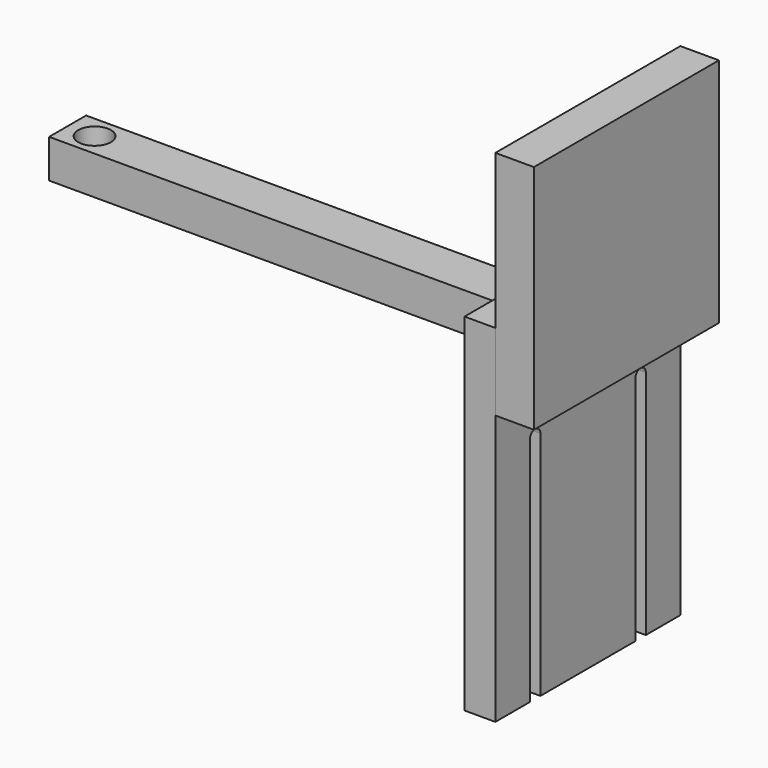
from build123d import *

# Parameters (mm, degrees)
F0_W     = 135
F0_H     = 12
F0_R     = 4.25
F1_DEPTH = 10
F0_W_2   = 5
F2_DEPTH = 60
F4_DEPTH = 5
F5_DEPTH = 3


with BuildPart() as f1:
    # F0 (on Top) → F1 (new body)
    with BuildSketch(Plane.XY):
        with Locations((-2.5, 0)):
            Rectangle(F0_W, F0_H)
        with Locations((-63, 0)):
            Circle(F0_R, mode=Mode.SUBTRACT)
    extrude(amount=F1_DEPTH)

    # F0 (on Top) → F2 (join)
    with BuildSketch(Plane.XY):
        Polygon((65, 30), (65, 6), (70, 6), (70, -6), (65, -6), (65, -30), (75, -30), (75, 30), align=None)
        with Locations((67.5, 0)):
            Rectangle(F0_W_2, F0_H)
    extrude(amount=F2_DEPTH)


with BuildPart() as f4:
    # F3 (on face) → F4 (new body)
    with BuildSketch(Plane(origin=(65, 0, 0), x_dir=(0, -1, 0), z_dir=(-1, 0, 0))):
        with BuildLine():
            Line((-6, 0), (-30, 0))
            Line((-30, 0), (-30, -70))
            Line((-30, -70), (-20, -70))
            Line((-20, -70), (-20, -10))
            ThreePointArc((-20, -10), (-17.1, -7.1), (-14.2, -10))
            Line((-14.2, -10), (-14.2, -70))
            Line((-14.2, -70), (14.2, -70))
            Line((14.2, -70), (14.2, -10))
            ThreePointArc((14.2, -10), (17.1, -7.1), (20, -10))
            Line((20, -10), (20, -70))
            Line((20, -70), (30, -70))
            Line((30, -70), (30, 0))
            Line((30, 0), (6, 0))
            Line((6, 0), (-6, 0))
        make_face()
        Polygon((-30, 20), (-30, 0), (-6, 0), (-6, 10), (-6, 20), align=None)
        Polygon((6, 10), (6, 0), (30, 0), (30, 20), (6, 20), align=None)
    extrude(amount=F4_DEPTH)

    # F3 (on face) + F4_face (on face) + F4_face1 (on face) → F5 (join)
    with BuildSketch(Plane(origin=(65, 0, 0), x_dir=(0, -1, 0), z_dir=(-1, 0, 0))):
        with BuildLine():
            Line((-20, -10), (-20, -70))
            Line((-20, -70), (-18.8, -70))
            Line((-18.8, -70), (-18.8, -10))
            ThreePointArc((-18.8, -10), (-17.1, -8.3), (-15.4, -10))
            Line((-15.4, -10), (-15.4, -70))
            Line((-15.4, -70), (-14.2, -70))
            Line((-14.2, -70), (-14.2, -10))
            ThreePointArc((-14.2, -10), (-17.1, -7.1), (-20, -10))
        make_face()
        with BuildLine():
            Line((18.8, -70), (20, -70))
            Line((20, -70), (20, -10))
            ThreePointArc((20, -10), (17.1, -7.1), (14.2, -10))
            Line((14.2, -10), (14.2, -70))
            Line((14.2, -70), (15.4, -70))
            Line((15.4, -70), (15.4, -10))
            ThreePointArc((15.4, -10), (17.1, -8.3), (18.8, -10))
            Line((18.8, -10), (18.8, -70))
        make_face()
        with BuildLine():
            Line((-6, 0), (-30, 0))
            Line((-30, 0), (-30, -70))
            Line((-30, -70), (-20, -70))
            Line((-20, -70), (-20, -10))
            ThreePointArc((-20, -10), (-17.1, -7.1), (-14.2, -10))
            Line((-14.2, -10), (-14.2, -70))
            Line((-14.2, -70), (14.2, -70))
            Line((14.2, -70), (14.2, -10))
            ThreePointArc((14.2, -10), (17.1, -7.1), (20, -10))
            Line((20, -10), (20, -70))
            Line((20, -70), (30, -70))
            Line((30, -70), (30, 0))
            Line((30, 0), (6, 0))
            Line((6, 0), (-6, 0))
        make_face()
    with BuildSketch(Plane(origin=(60, 0, -24.6369260479), x_dir=(0, -1, 0), z_dir=(-1, 0, 0))):
        with BuildLine():
            Line((20, 14.6369260479), (20, -45.3630739521))
            Line((20, -45.3630739521), (30, -45.3630739521))
            Line((30, -45.3630739521), (30, 44.6369260479))
            Line((30, 44.6369260479), (6, 44.6369260479))
            Line((6, 44.6369260479), (6, 24.6369260479))
            Line((6, 24.6369260479), (-6, 24.6369260479))
            Line((-6, 24.6369260479), (-6, 44.6369260479))
            Line((-6, 44.6369260479), (-30, 44.6369260479))
            Line((-30, 44.6369260479), (-30, -45.3630739521))
            Line((-30, -45.3630739521), (-20, -45.3630739521))
            Line((-20, -45.3630739521), (-20, 14.6369260479))
            ThreePointArc((-20, 14.6369260479), (-17.1, 17.5369260479), (-14.2, 14.6369260479))
            Line((-14.2, 14.6369260479), (-14.2, -45.3630739521))
            Line((-14.2, -45.3630739521), (14.2, -45.3630739521))
            Line((14.2, -45.3630739521), (14.2, 14.6369260479))
            ThreePointArc((14.2, 14.6369260479), (17.1, 17.5369260479), (20, 14.6369260479))
        make_face()
    with BuildSketch(Plane(origin=(65, 0, -24.6369260479), x_dir=(0, -1, 0), z_dir=(1, 0, 0))):
        with BuildLine():
            Line((20, 45.3630739521), (20, -14.6369260479))
            ThreePointArc((20, -14.6369260479), (17.1, -17.5369260479), (14.2, -14.6369260479))
            Line((14.2, -14.6369260479), (14.2, 45.3630739521))
            Line((14.2, 45.3630739521), (-14.2, 45.3630739521))
            Line((-14.2, 45.3630739521), (-14.2, -14.6369260479))
            ThreePointArc((-14.2, -14.6369260479), (-17.1, -17.5369260479), (-20, -14.6369260479))
            Line((-20, -14.6369260479), (-20, 45.3630739521))
            Line((-20, 45.3630739521), (-30, 45.3630739521))
            Line((-30, 45.3630739521), (-30, -44.6369260479))
            Line((-30, -44.6369260479), (-6, -44.6369260479))
            Line((-6, -44.6369260479), (-6, -24.6369260479))
            Line((-6, -24.6369260479), (6, -24.6369260479))
            Line((6, -24.6369260479), (6, -44.6369260479))
            Line((6, -44.6369260479), (30, -44.6369260479))
            Line((30, -44.6369260479), (30, 45.3630739521))
            Line((30, 45.3630739521), (20, 45.3630739521))
        make_face()
    extrude(amount=F5_DEPTH, dir=(-1, 0, 0))


solid = Compound([f1.part, f4.part])
